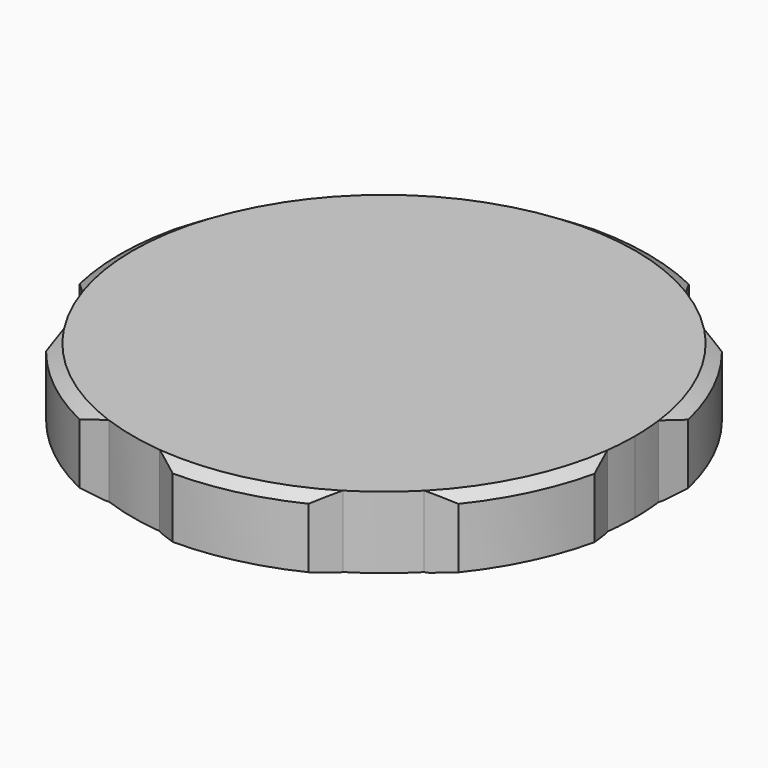
from build123d import *

# Parameters (mm, degrees)
F1_DEPTH   = 3.5
F2_SIZE2   = 0.357957
F2_SIZE    = 0.62
F3_SIZE2   = 0.549495
F3_SIZE    = 0.2
F3_2_SIZE2 = 0.549495
F3_2_SIZE  = 0.2
F3_3_SIZE2 = 0.549495
F3_3_SIZE  = 0.2
F3_4_SIZE2 = 0.549495
F3_4_SIZE  = 0.2
F3_5_SIZE2 = 0.549495
F3_5_SIZE  = 0.2
F3_6_SIZE2 = 0.549495
F3_6_SIZE  = 0.2
F3_7_SIZE2 = 0.549495
F3_7_SIZE  = 0.2


with BuildPart() as f1:
    # F0 (on Top) → F1 (new body)
    with BuildSketch(Plane.XY):
        with BuildLine():
            ThreePointArc((12.25, 0), (12.225309, 0.777384), (12.151335, 1.551633))
            ThreePointArc((12.151335, 1.551633), (11.036869, 5.315076), (8.789349, 8.532868))
            ThreePointArc((8.789349, 8.532868), (7.63775, 9.577436), (6.363117, 10.467724))
            ThreePointArc((6.363117, 10.467724), (2.725881, 11.942867), (-1.191196, 12.191946))
            ThreePointArc((-1.191196, 12.191946), (-2.725881, 11.942867), (-4.216657, 11.501404))
            ThreePointArc((-4.216657, 11.501404), (-7.63775, 9.577436), (-10.274746, 6.67024))
            ThreePointArc((-10.274746, 6.67024), (-11.036869, 5.315076), (-11.621203, 3.874293))
            ThreePointArc((-11.621203, 3.874293), (-12.25, 0), (-11.621203, -3.874293))
            ThreePointArc((-11.621203, -3.874293), (-11.036869, -5.315076), (-10.274746, -6.67024))
            ThreePointArc((-10.274746, -6.67024), (-7.63775, -9.577436), (-4.216657, -11.501404))
            ThreePointArc((-4.216657, -11.501404), (-2.725881, -11.942867), (-1.191196, -12.191946))
            ThreePointArc((-1.191196, -12.191946), (2.725881, -11.942867), (6.363117, -10.467724))
            ThreePointArc((6.363117, -10.467724), (7.63775, -9.577436), (8.789349, -8.532868))
            ThreePointArc((8.789349, -8.532868), (11.036869, -5.315076), (12.151335, -1.551633))
            ThreePointArc((12.151335, -1.551633), (12.225309, -0.777384), (12.25, 0))
        make_face()
        with BuildLine():
            Line((-4.216657, 11.501404), (-5.576969, 11.60444))
            ThreePointArc((-5.576969, 11.60444), (-8.027431, 10.06608), (-10.0725, 8.019374))
            Line((-10.0725, 8.019374), (-10.274746, 6.67024))
            ThreePointArc((-10.274746, 6.67024), (-7.63775, 9.577436), (-4.216657, 11.501404))
        make_face()
        with BuildLine():
            Line((6.363117, 10.467724), (5.595533, 11.595501))
            ThreePointArc((5.595533, 11.595501), (2.864957, 12.552197), (-0.010302, 12.874996))
            Line((-0.010302, 12.874996), (-1.191196, 12.191946))
            ThreePointArc((-1.191196, 12.191946), (2.725881, 11.942867), (6.363117, 10.467724))
        make_face()
        with BuildLine():
            Line((12.151335, 1.551633), (12.554485, 2.854912))
            ThreePointArc((12.554485, 2.854912), (11.599974, 5.586253), (10.059654, 8.035483))
            Line((10.059654, 8.035483), (8.789349, 8.532868))
            ThreePointArc((8.789349, 8.532868), (11.036869, 5.315076), (12.151335, 1.551633))
        make_face()
        with BuildLine():
            ThreePointArc((10.059654, -8.035483), (11.599974, -5.586253), (12.554485, -2.854912))
            Line((12.554485, -2.854912), (12.151335, -1.551633))
            ThreePointArc((12.151335, -1.551633), (11.036869, -5.315076), (8.789349, -8.532868))
            Line((8.789349, -8.532868), (10.059654, -8.035483))
        make_face()
        with BuildLine():
            Line((-11.621203, 3.874293), (-12.5499, 2.875))
            ThreePointArc((-12.5499, 2.875), (-12.875, 0), (-12.5499, -2.875))
            Line((-12.5499, -2.875), (-11.621203, -3.874293))
            ThreePointArc((-11.621203, -3.874293), (-12.25, 0), (-11.621203, 3.874293))
        make_face()
        with BuildLine():
            ThreePointArc((-10.0725, -8.019374), (-8.027431, -10.06608), (-5.576969, -11.60444))
            Line((-5.576969, -11.60444), (-4.216657, -11.501404))
            ThreePointArc((-4.216657, -11.501404), (-7.63775, -9.577436), (-10.274746, -6.67024))
            Line((-10.274746, -6.67024), (-10.0725, -8.019374))
        make_face()
        with BuildLine():
            ThreePointArc((-0.010302, -12.874996), (2.864957, -12.552197), (5.595533, -11.595501))
            Line((5.595533, -11.595501), (6.363117, -10.467724))
            ThreePointArc((6.363117, -10.467724), (2.725881, -11.942867), (-1.191196, -12.191946))
            Line((-1.191196, -12.191946), (-0.010302, -12.874996))
        make_face()
    extrude(amount=F1_DEPTH)

    # F2
    f2_edges = [f1.edges().sort_by_distance(p)[0] for p in [
        (-8.027431, -10.06608, 3.5),
        (-12.875, 0, 3.5),
        (-8.027431, 10.06608, 3.5),
        (2.864957, 12.552197, 3.5),
        (2.864957, -12.552197, 3.5),
        (11.599974, -5.586253, 3.5),
        (11.599974, 5.586253, 3.5),
    ]]
    f2_side = f1.faces().sort_by_distance((0, 0, 3.5))[0]
    chamfer(f2_edges, length=F2_SIZE, length2=F2_SIZE2, reference=f2_side)

    # F3
    f3_edges = [f1.edges().sort_by_distance(p)[0] for p in [
        (-8.027431, -10.06608, 0),
    ]]
    f3_side = f1.faces().sort_by_distance((-8.027431, -10.06608, 1.571021))[0]
    chamfer(f3_edges, length=F3_SIZE, length2=F3_SIZE2, reference=f3_side)

    # F3#2
    f3_2_edges = [f1.edges().sort_by_distance(p)[0] for p in [
        (2.864957, -12.552197, 0),
    ]]
    f3_2_side = f1.faces().sort_by_distance((2.864957, -12.552197, 1.571021))[0]
    chamfer(f3_2_edges, length=F3_2_SIZE, length2=F3_2_SIZE2, reference=f3_2_side)

    # F3#3
    f3_3_edges = [f1.edges().sort_by_distance(p)[0] for p in [
        (11.599974, -5.586253, 0),
    ]]
    f3_3_side = f1.faces().sort_by_distance((11.599974, -5.586253, 1.571021))[0]
    chamfer(f3_3_edges, length=F3_3_SIZE, length2=F3_3_SIZE2, reference=f3_3_side)

    # F3#4
    f3_4_edges = [f1.edges().sort_by_distance(p)[0] for p in [
        (11.599974, 5.586253, 0),
    ]]
    f3_4_side = f1.faces().sort_by_distance((11.599974, 5.586253, 1.571021))[0]
    chamfer(f3_4_edges, length=F3_4_SIZE, length2=F3_4_SIZE2, reference=f3_4_side)

    # F3#5
    f3_5_edges = [f1.edges().sort_by_distance(p)[0] for p in [
        (-12.875, 0, 0),
    ]]
    f3_5_side = f1.faces().sort_by_distance((-12.875, 0, 1.571021))[0]
    chamfer(f3_5_edges, length=F3_5_SIZE, length2=F3_5_SIZE2, reference=f3_5_side)

    # F3#6
    f3_6_edges = [f1.edges().sort_by_distance(p)[0] for p in [
        (-8.027431, 10.06608, 0),
    ]]
    f3_6_side = f1.faces().sort_by_distance((-8.027431, 10.06608, 1.571021))[0]
    chamfer(f3_6_edges, length=F3_6_SIZE, length2=F3_6_SIZE2, reference=f3_6_side)

    # F3#7
    f3_7_edges = [f1.edges().sort_by_distance(p)[0] for p in [
        (2.864957, 12.552197, 0),
    ]]
    f3_7_side = f1.faces().sort_by_distance((2.864957, 12.552197, 1.571021))[0]
    chamfer(f3_7_edges, length=F3_7_SIZE, length2=F3_7_SIZE2, reference=f3_7_side)


solid = f1.part
